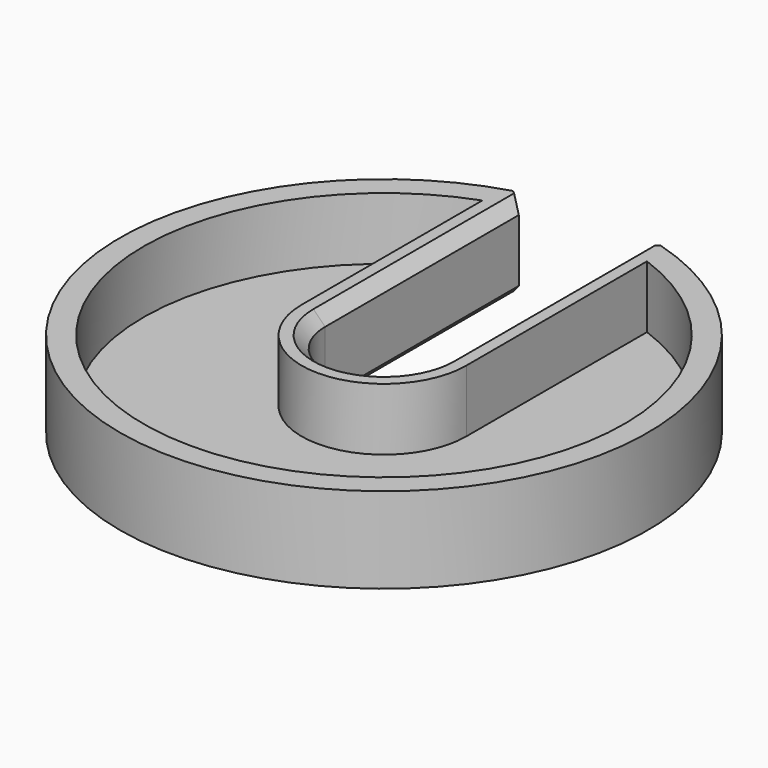
from build123d import *

# Parameters (mm, degrees)
F1_DEPTH    = 3.65
F2_T        = -1
F3_T1_DEPTH = 7.0190808226
F3_T3_DEPTH = 12.2237754854
F3_T6_ANGLE = 180
F3_T8_ANGLE = 180


# Not quite as in the source:
# - a fillet or chamfer that OpenCascade refuses, or shapes differently, is made with other operations: its cross-section is extruded or revolved along the edge and cut away or added


with BuildPart() as f1:
    # F0 (on Top) → F1 (new body)
    with BuildSketch(Plane.XY):
        with BuildLine():
            ThreePointArc((-2.5, 10.9379339914), (-6.9942261902, -8.773209219), (11.22, 0))
            ThreePointArc((11.22, 0), (8.773209219, 6.9942261902), (2.5, 10.9379339914))
            Line((2.5, 10.9379339914), (2.5, 0))
            ThreePointArc((2.5, 0), (0, -2.5), (-2.5, 0))
            Line((-2.5, 0), (-2.5, 10.9379339914))
        make_face()
    extrude(amount=F1_DEPTH)

    # F2
    f2_openings = [f1.faces().sort_by_distance(p)[0] for p in [
        (-6.797639, -8.52662, 3.65),
    ]]
    offset(amount=F2_T, openings=f2_openings)

    # F3: chamfer of 0.5 on 8 edges, made by hand

    # F3_s2 → F3_t1 (cut)
    with BuildSketch(Plane.XY.offset(-1.6845404113)):
        with BuildLine():
            Line((-3.1399253731, 10.7716882916), (-2.5, 10.2916665317))
            Line((-2.5, 10.2916665317), (-2.5, 10.9379339914))
            ThreePointArc((-2.5, 10.9379339914), (-2.8272189257, 10.857957135), (-3.1399253731, 10.7716882916))
        make_face()
        with BuildLine():
            Line((3.1399253731, 10.7716882916), (2.5, 10.2916665317))
            Line((2.5, 10.2916665317), (2.5, 10.9379339914))
            ThreePointArc((2.5, 10.9379339914), (2.8272189257, 10.857957135), (3.1399253731, 10.7716882916))
        make_face()
    extrude(amount=F3_T1_DEPTH, mode=Mode.SUBTRACT)

    # F3_s4 → F3_t3 (cut)
    with BuildSketch(Plane.XZ.offset(-12.2237754854)):
        Polygon((2.5, 0.5), (3, 0), (2.5, 0), align=None)
        Polygon((2.5, 3.15), (3, 3.65), (2.5, 3.65), align=None)
        Polygon((-2.5, 0.5), (-3, 0), (-2.5, 0), align=None)
        Polygon((-2.5, 3.15), (-3, 3.65), (-2.5, 3.65), align=None)
    extrude(amount=F3_T3_DEPTH, mode=Mode.SUBTRACT)

    # F3_s5 → F3_t6 (revolve, cut)
    with BuildSketch(Plane.XZ):
        Polygon((2.5, 3.15), (3, 3.65), (2.5, 3.65), align=None)
    revolve(axis=Axis((0, 0, 3.65), (0, 0, -1)), revolution_arc=F3_T6_ANGLE, mode=Mode.SUBTRACT)

    # F3_s7 → F3_t8 (revolve, cut)
    with BuildSketch(Plane.XZ):
        Polygon((2.5, 0.5), (3, 0), (2.5, 0), align=None)
    revolve(axis=Axis((0, 0, 0), (0, 0, -1)), revolution_arc=F3_T8_ANGLE, mode=Mode.SUBTRACT)


solid = f1.part
